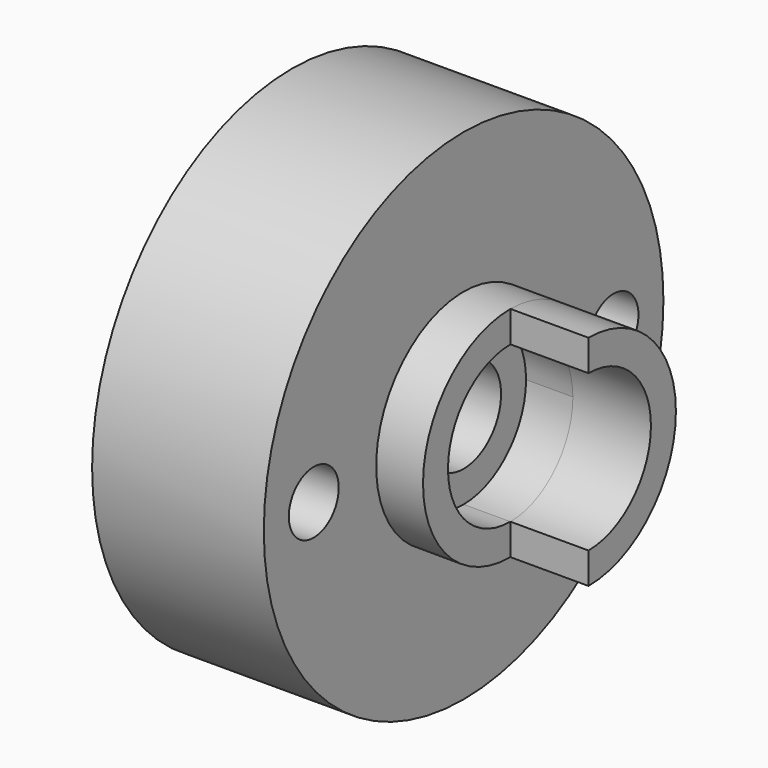
from build123d import *
from build123d import SkipClean  # not in build123d's __all__

# Parameters (mm, degrees)
F0_R            = 8
F1_DEPTH        = 5.5
F2_R            = 3.5
F3_DEPTH        = 1.5
F5_DEPTH        = 2.5
F7_DEPTH        = 1.5
F9_D            = 3
F10_R           = 1.5
F11_DEPTH       = 1
F13_D           = 2
F13_CSINK_D     = 3
F13_CSINK_ANGLE = 90


with BuildPart() as f1:
    # F0 (on Right) → F1 (new body)
    with BuildSketch(Plane.YZ):
        Circle(F0_R)
    extrude(amount=F1_DEPTH)

    # F2 (on face) → F3 (join)
    with BuildSketch(Plane.YZ.offset(5.5)):
        Circle(F2_R)
    extrude(amount=F3_DEPTH)

    # F4 (on face) → F5 (join)
    with BuildSketch(Plane.YZ.offset(7)):
        with BuildLine():
            Line((0, -2.5), (0, -3.5))
            ThreePointArc((0, -3.5), (2.4748737342, -2.4748737342), (3.5, 0))
            ThreePointArc((3.5, 0), (2.4748737342, 2.4748737342), (0, 3.5))
            Line((0, 3.5), (0, 2.5))
            ThreePointArc((0, 2.5), (2.5, 0), (0, -2.5))
        make_face()
    extrude(amount=F5_DEPTH)

    # F6 (on face) → F7 (cut)
    with BuildSketch(Plane.YZ.offset(7)):
        with BuildLine():
            ThreePointArc((0, -2.5), (1.767766953, -1.767766953), (2.5, 0))
            ThreePointArc((2.5, 0), (1.767766953, 1.767766953), (0, 2.5))
            ThreePointArc((0, 2.5), (-2.5, 0), (0, -2.5))
        make_face()
    with SkipClean():  # cleaning this boolean's faces spoils the solid; the shape is the same uncleaned
        extrude(amount=-F7_DEPTH, mode=Mode.SUBTRACT)

    # F9 (through all)
    with Locations(Plane.YZ.offset(5.5)):
        with Locations((0, 0)):
            Hole(F9_D / 2)

    # F10 (on face) → F11 (cut)
    with BuildSketch(Plane(origin=(0, 0, 0), x_dir=(0, -1, 0), z_dir=(-1, 0, 0))):
        with Locations((-6, 0)):
            Circle(F10_R)
        with Locations((6, 0)):
            Circle(F10_R)
    extrude(amount=-F11_DEPTH, mode=Mode.SUBTRACT)

    # F13 (through all)
    with Locations(Plane(origin=(1, 0, 0), x_dir=(0, -1, 0), z_dir=(-1, 0, 0))):
        with Locations((-6, 0), (6, 0)):
            CounterSinkHole(F13_D / 2, F13_CSINK_D / 2, counter_sink_angle=F13_CSINK_ANGLE)


solid = f1.part
